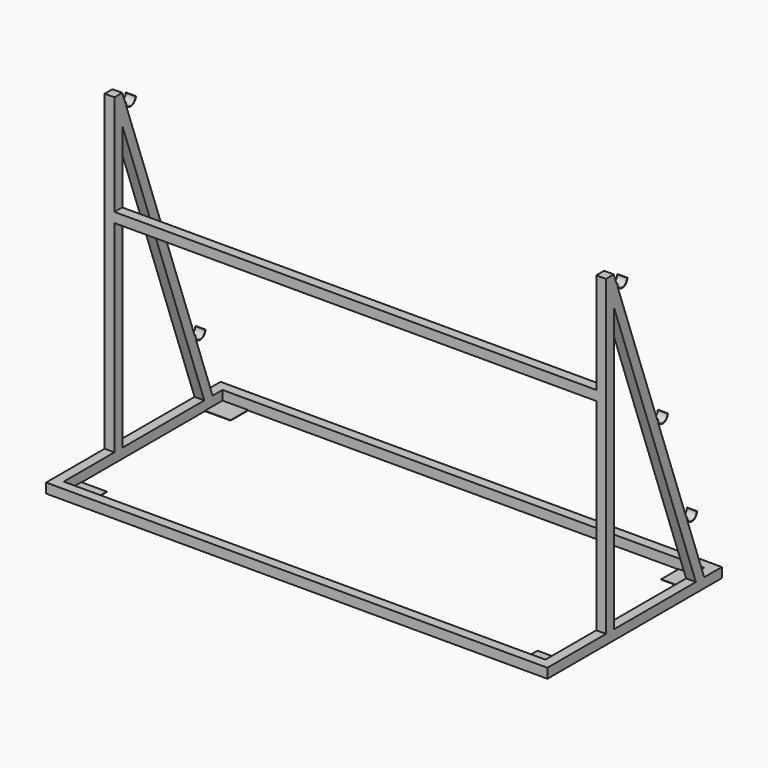
from build123d import *

# Parameters (mm, degrees)
F1_DEPTH  = 38.1
F4_W      = 38.1
F4_H      = 38.1
F5_DEPTH  = 1879.6
F6_W      = 38.1
F6_H      = 38.1
F7_DEPTH  = 1917.7
F9_DEPTH  = 38.1
F11_W     = 100.0125
F11_H     = 85.725
F12_DEPTH = 1.524


# Not quite as in the source:
# - an extrude ends at something that could not be found from the text; its depth is read off the source's solid


with BuildPart() as f1:
    # F0 (on Right) → F1 (new body)
    with BuildSketch(Plane.YZ):
        Polygon((-323.85, 38.1), (-323.85, 0), (527.05, 0), (527.05, 38.1), (440.5612396804, 38.1), (-0.0062959033, 1257.3), (-38.1, 1257.3), (-38.1, 38.1), align=None)
        Polygon((400.05, 38.1), (0, 38.1), (0, 1145.1742181533), align=None, mode=Mode.SUBTRACT)
    extrude(amount=F1_DEPTH)


with BuildPart() as f3_1:
    # F3: instance of F1
    add(f1.part.mirror(Plane.YZ.offset(-939.8)))


with BuildPart() as f1_1:
    add(f1.part)

    add(f3_1.part)  # F5 merges F3_1
    # F4 (on Right) → F5 (join, through all)
    with BuildSketch(Plane.YZ):
        with Locations((-304.8, 19.05)):
            Rectangle(F4_W, F4_H)
        with Locations((508, 19.05)):
            Rectangle(F4_W, F4_H)
    extrude(amount=-F5_DEPTH)

    # F6 (on Right) → F7 (join, through all)
    with BuildSketch(Plane.YZ):
        with Locations((-19.05, 844.55)):
            Rectangle(F6_W, F6_H)
    extrude(amount=-F7_DEPTH)

    # F11 (on face) → F12 (join)
    with BuildSketch(Plane(origin=(0, 0, 0), x_dir=(1, 0, 0), z_dir=(0, 0, -1))):
        with Locations((-50.00625, 242.8875)):
            Rectangle(F11_W, F11_H)
        with Locations((-50.00625, -446.0875)):
            Rectangle(F11_W, F11_H)
    extrude(amount=-F12_DEPTH)



with BuildPart() as f9:
    # F8 (on Right) → F9 (new body)
    with BuildSketch(Plane.YZ):
        with BuildLine():
            ThreePointArc((15.3689327039, 1219.2), (40.7689327039, 1193.8), (66.1689327039, 1219.2))
            Line((66.1689327039, 1219.2), (64.1369327039, 1219.2))
            ThreePointArc((64.1369327039, 1219.2), (40.7689327039, 1195.832), (17.4009327039, 1219.2))
            Line((17.4009327039, 1219.2), (15.3689327039, 1219.2))
        make_face()
    extrude(amount=F9_DEPTH)


with BuildPart() as f9b:
    # F8 (on Right) → F9, piece 2 (new body)
    with BuildSketch(Plane.YZ):
        with BuildLine():
            ThreePointArc((212.7064746841, 673.1), (238.1064746841, 647.7), (263.5064746841, 673.1))
            Line((263.5064746841, 673.1), (261.4744746841, 673.1))
            ThreePointArc((261.4744746841, 673.1), (238.1064746841, 649.732), (214.7384746841, 673.1))
            Line((214.7384746841, 673.1), (212.7064746841, 673.1))
        make_face()
    extrude(amount=F9_DEPTH)


with BuildPart() as f9c:
    # F8 (on Right) → F9, piece 3 (new body)
    with BuildSketch(Plane.YZ):
        with BuildLine():
            ThreePointArc((354.9730747163, 279.4), (380.3730747163, 254), (405.7730747163, 279.4))
            Line((405.7730747163, 279.4), (403.7410747163, 279.4))
            ThreePointArc((403.7410747163, 279.4), (380.3730747163, 256.032), (357.0050747163, 279.4))
            Line((357.0050747163, 279.4), (354.9730747163, 279.4))
        make_face()
    extrude(amount=F9_DEPTH)


with BuildPart() as f10_1:
    # F10: instance of F9
    add(f9.part.mirror(Plane.YZ.offset(-939.8)))


with BuildPart() as f10_2:
    # F10: instance of F9b
    add(f9b.part.mirror(Plane.YZ.offset(-939.8)))


with BuildPart() as f10_3:
    # F10: instance of F9c
    add(f9c.part.mirror(Plane.YZ.offset(-939.8)))


with BuildPart() as f1_2:
    add(f1_1.part)

    add(f9.part)  # F13 merges F9

    add(f9b.part)  # F13 merges F9b

    add(f9c.part)  # F13 merges F9c

    add(f10_1.part)  # F13 merges F10_1

    add(f10_2.part)  # F13 merges F10_2

    add(f10_3.part)  # F13 merges F10_3
    # F13: F1 across plane
    add(f1_1.part.mirror(Plane.YZ.offset(-939.8)))


solid = f1_2.part
